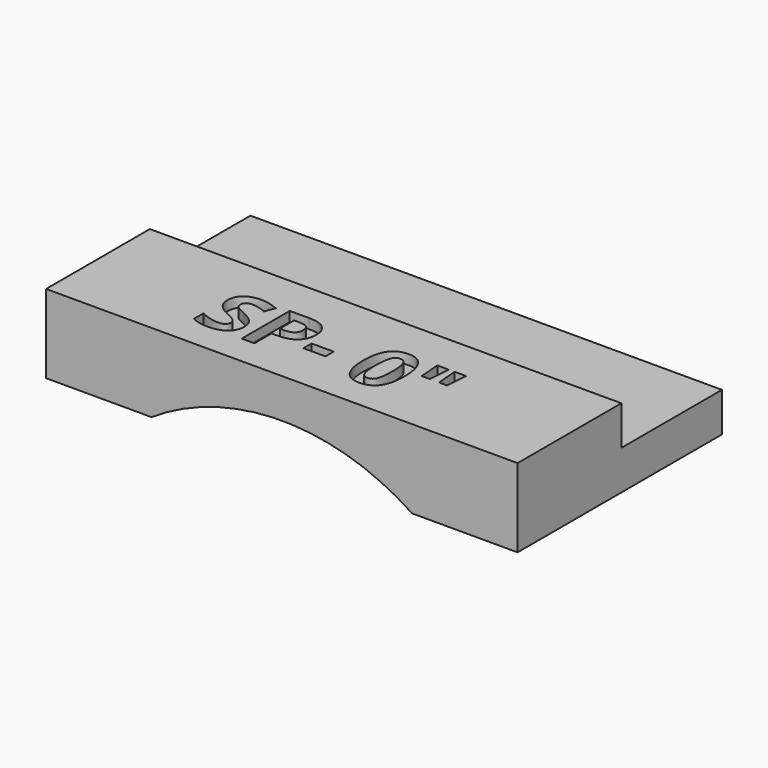
from build123d import *

# Parameters (mm, degrees)
F1_DEPTH     = 39.6875
F2_W         = 152.4
F2_H         = 25.4
F3_DEPTH     = 42.8625
F4_W         = 152.4
F4_H         = 12.7
F5_DEPTH     = 40.64
F6_TEXT_SIZE = 27.1839464883
F7_DEPTH     = 3.175


# Not quite as in the source:
# - Text() gives the source's letters only with a copy of the font that has no kerning and outlines rounded to 1/6400 em; it was checked with that copy


with BuildPart() as f1:
    # F0 (on Front) → F1 (new body)
    with BuildSketch(Plane.XZ):
        with BuildLine():
            Line((0, 25.4), (0, 0))
            Line((0, 0), (34.0788651625, 0))
            ThreePointArc((34.0788651625, 0), (76.2, 12.7), (118.3211348375, 0))
            Line((118.3211348375, 0), (152.4, 0))
            Line((152.4, 0), (152.4, 25.4))
            Line((152.4, 25.4), (0, 25.4))
        make_face()
    extrude(amount=F1_DEPTH)

    # F2 (on face) → F3 (join)
    with BuildSketch(Plane(origin=(0, 0, 0), x_dir=(-1, 0, 0), z_dir=(0, 1, 0))):
        with Locations((-76.2, 12.7)):
            Rectangle(F2_W, F2_H)
    extrude(amount=F3_DEPTH)

    # F4 (on face) → F5 (cut)
    with BuildSketch(Plane(origin=(0, 42.8625, 0), x_dir=(-1, 0, 0), z_dir=(0, 1, 0))):
        with Locations((-76.2, 19.05)):
            Rectangle(F4_W, F4_H)
    extrude(amount=-F5_DEPTH, mode=Mode.SUBTRACT)

    # F6 (on face) → F7 (cut)
    with BuildSketch(Plane.XY.offset(25.4)):
        with Locations((38.1, -30.0499414716)):
            Text('SP- 0"', F6_TEXT_SIZE, font='Open Sans', font_style=FontStyle.BOLD, text_align=(TextAlign.LEFT, TextAlign.BOTTOM))
    extrude(amount=-F7_DEPTH, mode=Mode.SUBTRACT)


solid = f1.part
